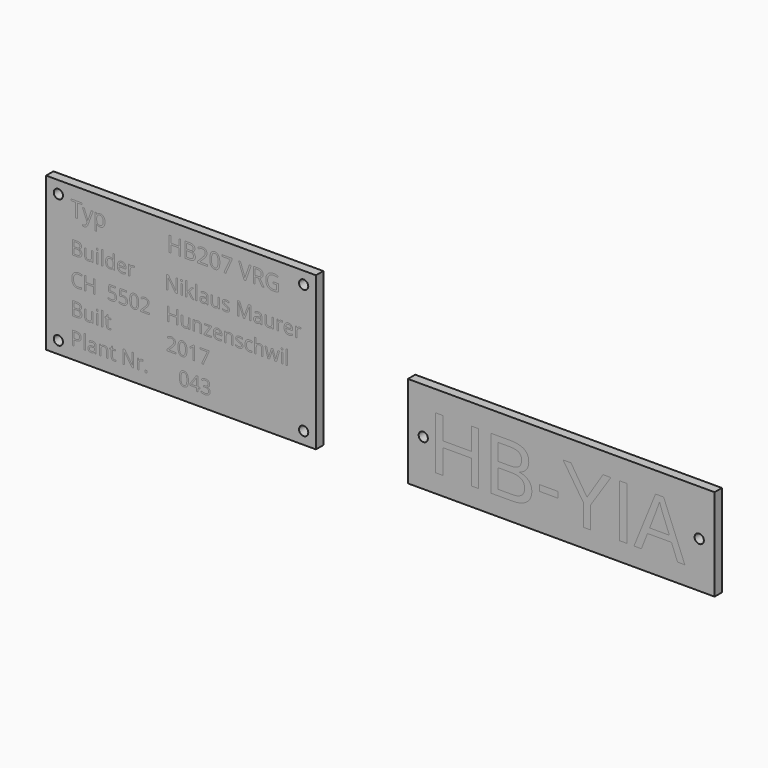
from build123d import *

# Parameters (mm, degrees)
F0_W           = 88
F0_H           = 50
F0_R           = 1.5
F1_DEPTH       = 3
F0_W_2         = 100
F0_H_2         = 30
F2_TEXT_SIZE   = 25
F2_TEXT_SIZE_2 = 6.9444444444
F2_TEXT_SIZE_3 = 6.25
F3_DEPTH       = 1.5


# Not quite as in the source:
# - Text() gives the source's letters only with a copy of the font that has no kerning and outlines rounded to 1/6400 em; it was checked with that copy


with BuildPart() as f1:
    # F0 (on Front) → F1 (new body)
    with BuildSketch(Plane.XZ):
        with Locations((-44, 25)):
            Rectangle(F0_W, F0_H)
        with Locations((-84, 4)):
            Circle(F0_R, mode=Mode.SUBTRACT)
        with Locations((-4, 4)):
            Circle(F0_R, mode=Mode.SUBTRACT)
        with Locations((-84, 46)):
            Circle(F0_R, mode=Mode.SUBTRACT)
        with Locations((-4, 46)):
            Circle(F0_R, mode=Mode.SUBTRACT)
    extrude(amount=F1_DEPTH)


with BuildPart() as f1b:
    # F0 (on Front) → F1, piece 2 (new body)
    with BuildSketch(Plane.XZ):
        with Locations((80, 15)):
            Rectangle(F0_W_2, F0_H_2)
        with Locations((35, 15)):
            Circle(F0_R, mode=Mode.SUBTRACT)
        with Locations((125, 15)):
            Circle(F0_R, mode=Mode.SUBTRACT)
    extrude(amount=F1_DEPTH)


with BuildPart() as f3:
    # F2 (on face) → F3 (new body)
    with BuildSketch(Plane.XZ.offset(3)):
        with Locations((37, 6)):
            Text('HB-YIA', F2_TEXT_SIZE, font='Arimo', text_align=(TextAlign.LEFT, TextAlign.BOTTOM))
        with Locations((-80, 41)):
            Text('Typ           HB207 VRG', F2_TEXT_SIZE_2, font='Open Sans', text_align=(TextAlign.LEFT, TextAlign.BOTTOM))
        with Locations((-80, 30)):
            Text('Builder      Niklaus Maurer', F2_TEXT_SIZE_3, font='Open Sans', text_align=(TextAlign.LEFT, TextAlign.BOTTOM))
        with Locations((-80, 21)):
            Text('CH  5502   Hunzenschwil', F2_TEXT_SIZE_3, font='Open Sans', text_align=(TextAlign.LEFT, TextAlign.BOTTOM))
        with Locations((-80, 12.5)):
            Text('Built           2017', F2_TEXT_SIZE_3, font='Open Sans', text_align=(TextAlign.LEFT, TextAlign.BOTTOM))
        with Locations((-80, 4)):
            Text('Plant Nr.      043', F2_TEXT_SIZE_3, font='Open Sans', text_align=(TextAlign.LEFT, TextAlign.BOTTOM))
    extrude(amount=-F3_DEPTH)


solid = Compound([f1.part, f1b.part, f3.part])
